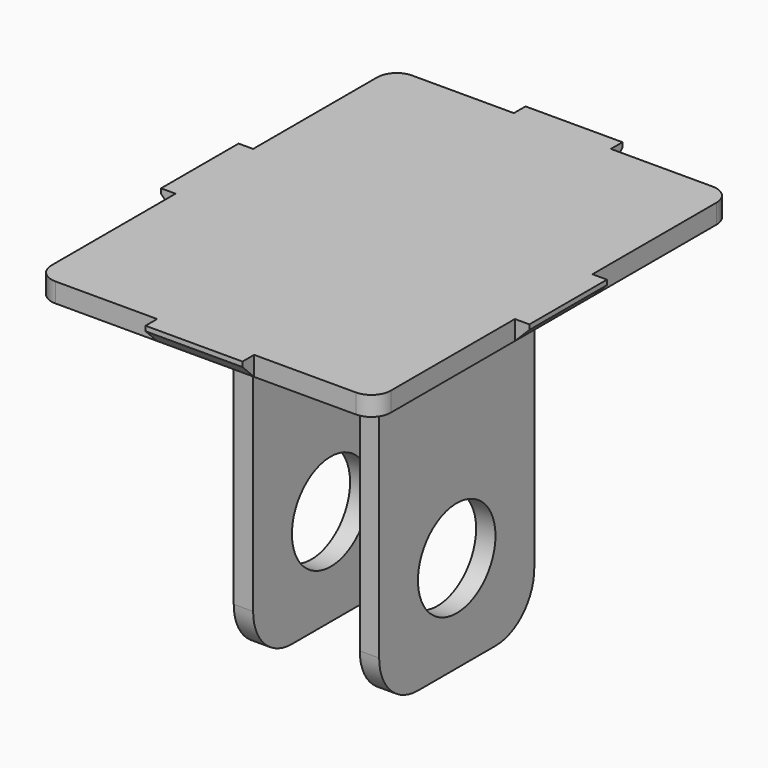
from build123d import *

# Parameters (mm, degrees)
F1_DEPTH = 20
F3_D     = 10
F3_DEPTH = 45
F3_TIP   = 3.0043030951
F4_W     = 15
F4_H     = 20
F5_DEPTH = 2
F6_DEPTH = 26.501
F7_SIZE  = 1.5


with BuildPart() as f1:
    # F0 (on Front) → F1 (new body)
    with BuildSketch(Plane.XZ):
        with BuildLine():
            Line((7.5, 35), (0, 35))
            Line((0, 35), (-7.5, 35))
            Line((-7.5, 35), (-7.5, 0))
            Line((-7.5, 0), (-5.5, 0))
            Line((-5.5, 0), (-5.5, 31))
            ThreePointArc((-5.5, 31), (-4.9142135624, 32.4142135624), (-3.5, 33))
            Line((-3.5, 33), (0, 33))
            Line((0, 33), (3.5, 33))
            ThreePointArc((3.5, 33), (4.9142135624, 32.4142135624), (5.5, 31))
            Line((5.5, 31), (5.5, 0))
            Line((5.5, 0), (7.5, 0))
            Line((7.5, 0), (7.5, 35))
        make_face()
    extrude(amount=F1_DEPTH)

    # F3
    with Locations(Plane(origin=(-7.5, 0, 0), x_dir=(0, -1, 0), z_dir=(-1, 0, 0))):
        with Locations((10, 10)):
            Hole(F3_D / 2, depth=F3_DEPTH)
            with Locations((0, 0, -(F3_DEPTH + F3_TIP / 2))):  # 118° drill point
                Cone(0, F3_D / 2, F3_TIP, mode=Mode.SUBTRACT)

    # F4 (on face) → F5 (join)
    with BuildSketch(Plane.XY.offset(35)):
        with BuildLine():
            Line((5, -33), (15.5, -33))
            ThreePointArc((15.5, -33), (16.9142135624, -32.4142135624), (17.5, -31))
            Line((17.5, -31), (17.5, -15))
            Line((17.5, -15), (17.5, -5))
            Line((17.5, -5), (17.5, 11))
            ThreePointArc((17.5, 11), (16.9142135624, 12.4142135624), (15.5, 13))
            Line((15.5, 13), (5, 13))
            Line((5, 13), (0, 13))
            Line((0, 13), (-5, 13))
            Line((-5, 13), (-15.5, 13))
            ThreePointArc((-15.5, 13), (-16.9142135624, 12.4142135624), (-17.5, 11))
            Line((-17.5, 11), (-17.5, -5))
            Line((-17.5, -5), (-17.5, -10))
            Line((-17.5, -10), (-17.5, -15))
            Line((-17.5, -15), (-17.5, -31))
            ThreePointArc((-17.5, -31), (-16.9142135624, -32.4142135624), (-15.5, -33))
            Line((-15.5, -33), (-5, -33))
            Line((-5, -33), (5, -33))
        make_face()
        with Locations((0, -10)):
            Rectangle(F4_W, F4_H, mode=Mode.SUBTRACT)
        Polygon((5, -34.5), (5, -33), (-5, -33), (-5, -34.5), (0, -34.5), align=None)
        Polygon((17.5, -5), (17.5, -15), (19, -15), (19, -10), (19, -5), align=None)
        Polygon((-19, -15), (-17.5, -15), (-17.5, -10), (-17.5, -5), (-19, -5), (-19, -10), align=None)
        Polygon((0, 13), (5, 13), (5, 14.5), (0, 14.5), (-5, 14.5), (-5, 13), align=None)
        with Locations((0, -10)):
            Rectangle(F4_W, F4_H)
    extrude(amount=F5_DEPTH)

    # F2 (on face) → F6 (cut, through all)
    with BuildSketch(Plane(origin=(-7.5, 0, 0), x_dir=(0, -1, 0), z_dir=(-1, 0, 0))):
        with BuildLine():
            Line((20, 0), (20, 5))
            ThreePointArc((20, 5), (18.5355339059, 1.4644660941), (15, 0))
            Line((15, 0), (20, 0))
        make_face()
        with BuildLine():
            ThreePointArc((5, 0), (1.4644660941, 1.4644660941), (0, 5))
            Line((0, 5), (0, 0))
            Line((0, 0), (5, 0))
        make_face()
    extrude(amount=-F6_DEPTH, mode=Mode.SUBTRACT)

    # F7
    f7_edges = [f1.edges().sort_by_distance(p)[0] for p in [
        (-19, -10, 35),
        (0, 14.5, 35),
        (19, -10, 35),
        (0, -34.5, 35),
    ]]
    chamfer(f7_edges, length=F7_SIZE)


solid = f1.part
